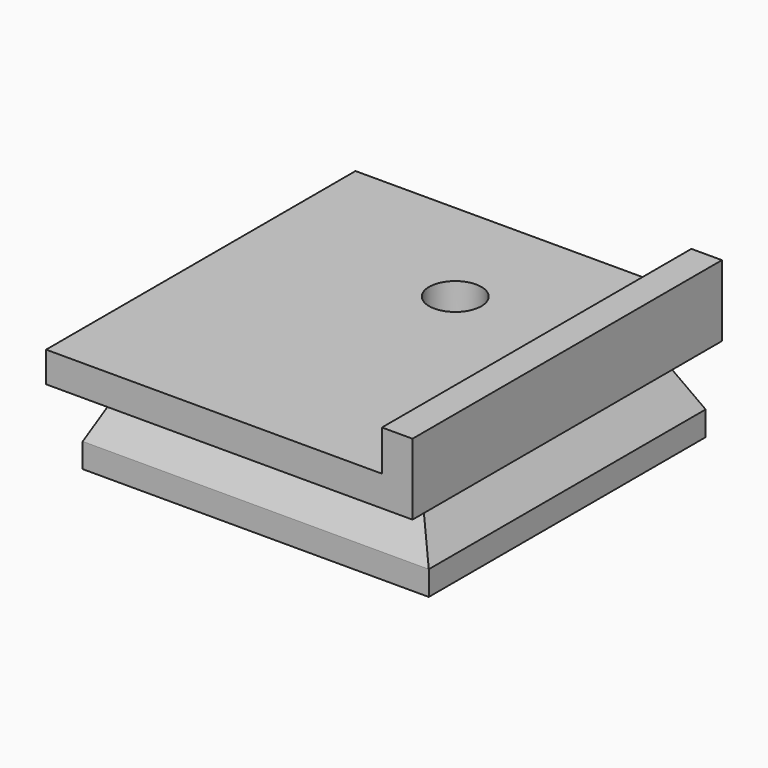
from build123d import *

# Parameters (mm, degrees)
F0_W      = 43.18
F0_H      = 43.18
F3_DEPTH  = 3.048
F3_FACE_W = 43.18
F3_FACE_H = 43.18
F2_W      = 36.83
F2_H      = 36.83
F5_R      = 7.62
F6_DEPTH  = 3.81
F7_R      = 3.2639
F8_DEPTH  = 25.4
F9_W      = 36.83
F9_H      = 36.83
F9_W_2    = 43.18
F9_H_2    = 2.54
F9_R      = 3.2639
F10_DEPTH = 3.81
F11_W     = 3.81
F11_H     = 48.26
F12_DEPTH = 5.08


# Not quite as in the source:
# - a feature names something its author has since deleted; it is built from what else it names


with BuildPart() as f3:
    # F0 (on Top) → F3 (new body)
    with BuildSketch(Plane.XY):
        Rectangle(F0_W, F0_H)
    extrude(amount=-F3_DEPTH)

    # F3_face (on face) → F4 section 0
    with BuildSketch(Plane.XY):
        Rectangle(F3_FACE_W, F3_FACE_H)
    # F2 (on offset) → F4 section 1
    with BuildSketch(Plane.XY.offset(6.477)):
        with Locations((-0.127, -0.127)):
            Rectangle(F2_W, F2_H)
    loft()

    # F5 (on face) → F6 (cut)
    with BuildSketch(Plane(origin=(0, 0, -3.048), x_dir=(1, 0, 0), z_dir=(0, 0, -1))):
        with Locations((0, -9.525)):
            Circle(F5_R)
    extrude(amount=-F6_DEPTH, mode=Mode.SUBTRACT)

    # F7 (on face) → F8 (cut)
    with BuildSketch(Plane(origin=(0, 0, 0.762), x_dir=(1, 0, 0), z_dir=(0, 0, -1))):
        with Locations((0, -9.525)):
            Circle(F7_R)
    extrude(amount=-F8_DEPTH, mode=Mode.SUBTRACT)

    # F9 (on face) → F10 (join)
    with BuildSketch(Plane.XY.offset(6.477)):
        Polygon((-21.59, 24.13), (-21.59, 21.59), (-21.59, -21.59), (21.59, -21.59), (21.59, 21.59), (21.59, 24.13), align=None)
        with Locations((-0.127, -0.127)):
            Rectangle(F9_W, F9_H, mode=Mode.SUBTRACT)
        Polygon((-21.59, -21.59), (-21.59, 21.59), (-21.59, 24.13), (-24.13, 24.13), (-24.13, -24.13), (-21.59, -24.13), align=None)
        with Locations((0, -22.86)):
            Rectangle(F9_W_2, F9_H_2)
        with Locations((-0.127, -0.127)):
            Rectangle(F9_W, F9_H)
        with Locations((0, 9.525)):
            Circle(F9_R, mode=Mode.SUBTRACT)
    extrude(amount=F10_DEPTH)

    # F11 (on face) → F12 (join)
    with BuildSketch(Plane.XY.offset(10.287)):
        with Locations((19.685, 0)):
            Rectangle(F11_W, F11_H)
    extrude(amount=F12_DEPTH)


solid = f3.part
